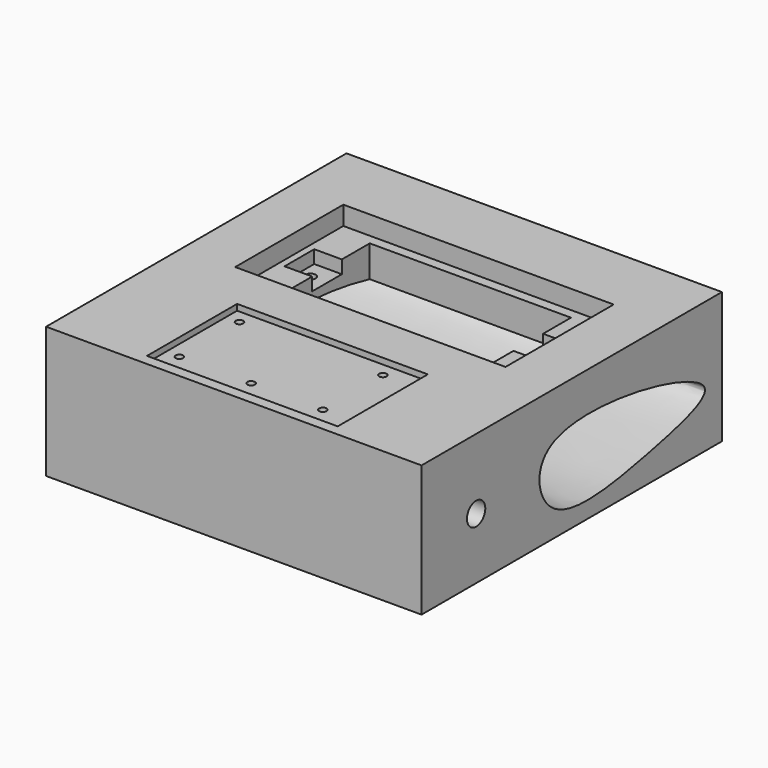
from build123d import *

# Parameters (mm, degrees)
F0_W      = 127
F0_H      = 127
F1_DEPTH  = 44.45
F2_W      = 64.516
F2_H      = 38.1
F3_DEPTH  = 2.032
F4_R      = 1.27
F5_DEPTH  = 12.192
F6_R      = 1.27
F7_DEPTH  = 12.192
F9_DEPTH  = 127
F10_W     = 91.44
F10_H     = 45.72
F11_DEPTH = 6.35
F12_W     = 68.072
F12_H     = 38.876
F13_DEPTH = 13.87
F14_W     = 9.35
F14_H     = 12.54
F15_DEPTH = 4.41
F16_R     = 1.74
F17_DEPTH = 8.4
F18_W     = 50
F18_H     = 23
F19_DEPTH = 52.59892
F20_W     = 31
F20_H     = 23
F21_DEPTH = 30
F22_R     = 3.875
F23_DEPTH = 10.4


with BuildPart() as f1:
    # F0 (on Top) → F1 (new body)
    with BuildSketch(Plane.XY):
        Rectangle(F0_W, F0_H)
    extrude(amount=F1_DEPTH)

    # F2 (on face) → F3 (cut)
    with BuildSketch(Plane.XY.offset(44.45)):
        with Locations((0, -40.8426690847)):
            Rectangle(F2_W, F2_H)
    extrude(amount=-F3_DEPTH, mode=Mode.SUBTRACT)

    # F4 (on face) → F5 (cut)
    with BuildSketch(Plane.XY.offset(42.418)):
        with Locations((20.828, -26.4916690847)):
            Circle(F4_R)
        with Locations((20.828, -51.8916690847)):
            Circle(F4_R)
        with Locations((-3.429, -51.8916690847)):
            Circle(F4_R)
        with Locations((-3.429, -26.4916690847)):
            Circle(F4_R)
        with Locations((-27.686, -26.4916690847)):
            Circle(F4_R)
        with Locations((-27.686, -51.8916690847)):
            Circle(F4_R)
    extrude(amount=-F5_DEPTH, mode=Mode.SUBTRACT)

    # F6 (on face) → F7 (join, through all)
    with BuildSketch(Plane.XY.offset(30.226)):
        with Locations((-3.429, -26.4916690847)):
            Circle(F6_R)
    extrude(amount=F7_DEPTH)

    # F8 (on face) → F9 (cut, through all)
    with BuildSketch(Plane.YZ.offset(63.5)):
        with BuildLine():
            add(Edge.make_bspline(
                [(-9.0976032104, 10.0759316516), (-14.4431789893, 14.8498555161), (-18.9998192848, 41.3407976718), (79.8789980532, 20.1886498245), (28.9220234676, 7.8572214413), (-0.9875973505, 2.8332038113), (-9.0976032104, 10.0759316516)],
                knots=[0, 0, 0, 0, 0.1786168384, 0.5173503637, 0.7290126141, 1, 1, 1, 1], degree=3))
        make_face()
    extrude(amount=-F9_DEPTH, mode=Mode.SUBTRACT)

    # F10 (on face) → F11 (cut)
    with BuildSketch(Plane.XY.offset(44.45)):
        with Locations((-0.09, 17.2031538572)):
            Rectangle(F10_W, F10_H)
    extrude(amount=-F11_DEPTH, mode=Mode.SUBTRACT)

    # F12 (on face) → F13 (cut)
    with BuildSketch(Plane.XY.offset(38.1)):
        with Locations((-0.124, 17.2251538572)):
            Rectangle(F12_W, F12_H)
    extrude(amount=-F13_DEPTH, mode=Mode.SUBTRACT)

    # F14 (on face) → F15 (cut)
    with BuildSketch(Plane.XY.offset(38.1)):
        with Locations((-38.835, 18.6161745679)):
            Rectangle(F14_W, F14_H)
        with Locations((38.565, 18.6161745679)):
            Rectangle(F14_W, F14_H)
    extrude(amount=-F15_DEPTH, mode=Mode.SUBTRACT)

    # F16 (on face) → F17 (cut)
    with BuildSketch(Plane.XY.offset(33.69)):
        with Locations((39.5, 18.6161745679)):
            Circle(F16_R)
        with Locations((-39.77, 18.657527864)):
            Circle(F16_R)
    extrude(amount=-F17_DEPTH, mode=Mode.SUBTRACT)

    # F18 (on Front) → F19 (cut)
    with BuildSketch(Plane.XZ):
        with Locations((-1.5, 20.0853766873)):
            Rectangle(F18_W, F18_H)
    extrude(amount=F19_DEPTH, mode=Mode.SUBTRACT)

    # F20 (on face) → F21 (cut)
    with BuildSketch(Plane(origin=(23.5, 0, 0), x_dir=(0, -1, 0), z_dir=(-1, 0, 0))):
        with Locations((37.09892, 20.0853766873)):
            Rectangle(F20_W, F20_H)
    extrude(amount=-F21_DEPTH, mode=Mode.SUBTRACT)

    # F22 (on face) → F23 (cut)
    with BuildSketch(Plane(origin=(53.5, 0, 0), x_dir=(0, -1, 0), z_dir=(-1, 0, 0))):
        with Locations((40.42392, 20.6998754293)):
            Circle(F22_R)
    extrude(amount=-F23_DEPTH, mode=Mode.SUBTRACT)


solid = f1.part
